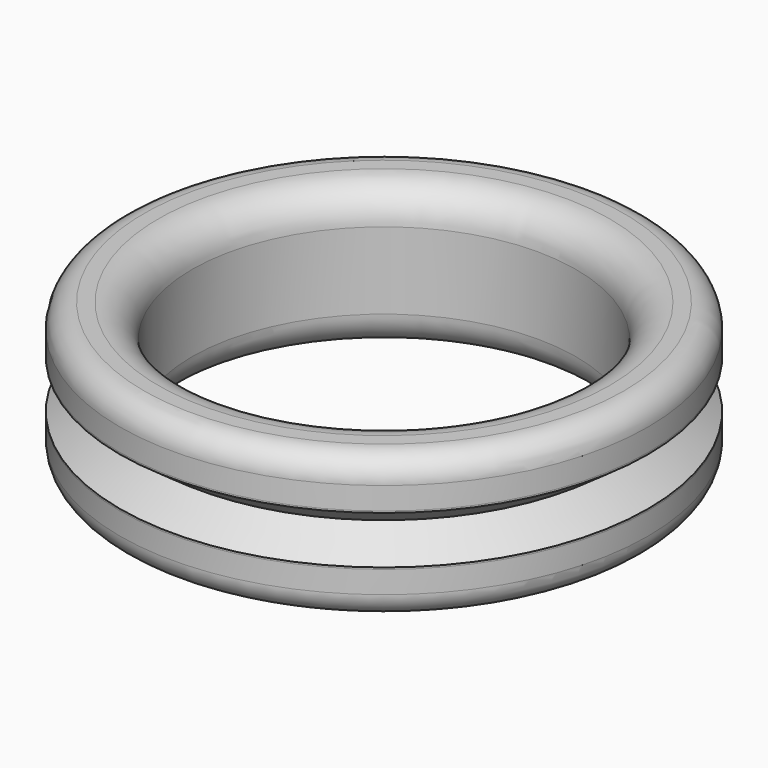
from build123d import *

# Parameters (mm, degrees)
F0_R     = 13.97
F0_R_2   = 10.16
F1_DEPTH = 3.81
F4_R     = 1.778
F5_R     = 1.27


# Not quite as in the source:
# - a fillet or chamfer that OpenCascade refuses, or shapes differently, is made with other operations: its cross-section is extruded or revolved along the edge and cut away or added


with BuildPart() as f1:
    # F0 (on Top) → F1 (new body, symmetric)
    with BuildSketch(Plane.XY):
        Circle(F0_R)
        Circle(F0_R_2, mode=Mode.SUBTRACT)
    extrude(amount=F1_DEPTH, both=True)

    # F2 (on Front) → F3 (revolve, cut)
    with BuildSketch(Plane.XZ):
        Polygon((-13.9681100845, -1.272341935), (-13.9681100845, 0), (-13.9681100845, 1.2655239552), (-15.1224341244, 1.2655239552), (-15.1224341244, -1.272341935), align=None)
        Polygon((-13.9681100845, 1.2655239552), (-13.9681100845, 0), (-13.9681100845, -1.272341935), (-12.1866818517, 0), align=None)
    revolve(axis=Axis((0, 0, 3.81), (0, 0, 1)), mode=Mode.SUBTRACT)

    # F4
    f4_edges = [f1.edges().sort_by_distance(p)[0] for p in [
        (-10.16, 0, 3.81),
        (10.16, 0, 0),
        (-10.16, 0, -3.81),
    ]]
    fillet(f4_edges, radius=F4_R)

    # F5
    f5_edges = [f1.edges().sort_by_distance(p)[0] for p in [
        (-13.97, 0, 3.81),
        (-13.97, 0, -3.81),
    ]]
    fillet(f5_edges, radius=F5_R)

    # F6: fillet of radius 2.286 on 2 edges, made by hand

    # F6_s1 → F6_t2 (revolve, cut)
    with BuildSketch(Plane.XZ):
        with BuildLine():
            ThreePointArc((13.97, -1.3652780514), (13.9695274723, -1.318800386), (13.9681100845, -1.272341935))
            Line((13.9681100845, -1.272341935), (13.97, -1.272341935))
            Line((13.97, -1.272341935), (13.97, -1.3652780514))
        make_face()
    revolve(axis=Axis((0, 0, -1.272341935), (0, 0, 1)), mode=Mode.SUBTRACT)

    # F6_s3 → F6_t4 (revolve, cut)
    with BuildSketch(Plane.XZ):
        with BuildLine():
            ThreePointArc((13.9681100845, 1.2655239552), (13.9695274723, 1.3119824063), (13.97, 1.3584600716))
            Line((13.97, 1.3584600716), (13.97, 1.2655239552))
            Line((13.97, 1.2655239552), (13.9681100845, 1.2655239552))
        make_face()
    revolve(axis=Axis((0, 0, 1.2655239552), (0, 0, 1)), mode=Mode.SUBTRACT)


solid = f1.part
